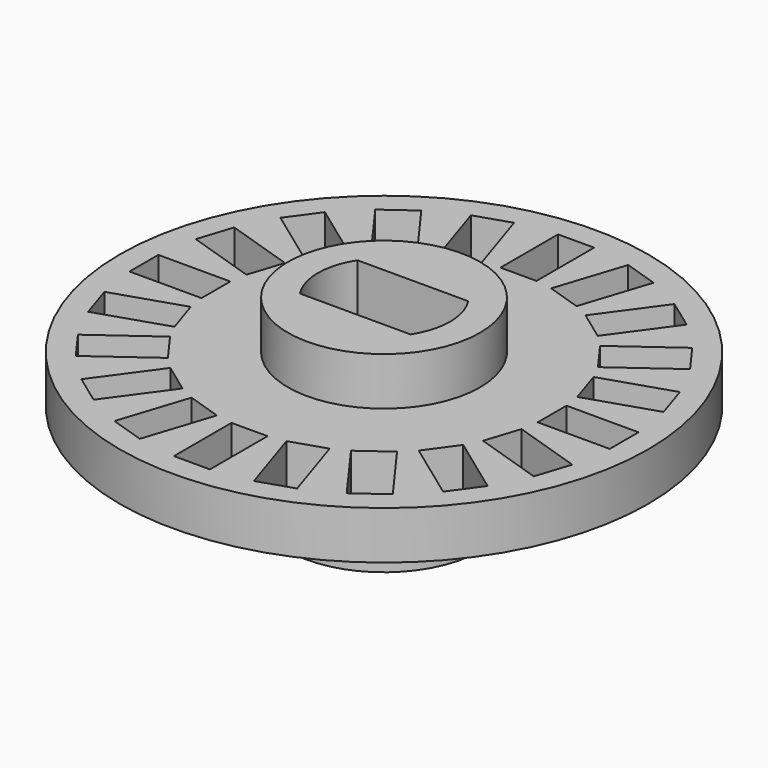
from build123d import *

# Parameters (mm, degrees)
F0_R            = 11
F1_DEPTH        = 2
F2_W            = 3
F2_H            = 1.5
F3_DEPTH        = 2
F3_COPIES_COUNT = 20
F4_R            = 4
F5_DEPTH        = 4
F5_DEPTH_BACK   = 4
F7_DEPTH        = 9


# Not quite as in the source:
# - a pattern or mirror of a feature is missing from the dataset's text; its kind, count and spacing are read off the source's solid


with BuildPart() as f1:
    # F0 (on Top) → F1 (new body)
    with BuildSketch(Plane.XY):
        Circle(F0_R)
    extrude(amount=F1_DEPTH)

    # F2 (on face) → F3 (cut)
    with BuildSketch(Plane.XY.offset(2)):
        with Locations((8.5, 0)):
            Rectangle(F2_W, F2_H)
    f3 = extrude(amount=-F3_DEPTH, mode=Mode.SUBTRACT)

    # F3_copies: F3 ×20 about axis
    f3_copies_axis = Axis((0, 0, 0), (0, 0, 1))
    for i in range(1, F3_COPIES_COUNT):
        add(f3.rotate(f3_copies_axis, i * 360 / F3_COPIES_COUNT), mode=Mode.SUBTRACT)

    # F4 (on face) → F5 (join, two sides)
    with BuildSketch(Plane(origin=(0, 0, 0), x_dir=(1, 0, 0), z_dir=(0, 0, -1))) as f5_sk:
        Circle(F4_R)
    extrude(amount=F5_DEPTH)
    extrude(f5_sk.sketch, amount=-F5_DEPTH_BACK)

    # F6 (on face) → F7 (cut)
    with BuildSketch(Plane.XY.offset(4)):
        with BuildLine():
            Line((-2.3048861143, -1.5), (2.3048861143, -1.5))
            ThreePointArc((2.3048861143, -1.5), (2.75, 0), (2.3048861143, 1.5))
            Line((2.3048861143, 1.5), (-2.3048861143, 1.5))
            ThreePointArc((-2.3048861143, 1.5), (-2.75, 0), (-2.3048861143, -1.5))
        make_face()
    extrude(amount=-F7_DEPTH, mode=Mode.SUBTRACT)


solid = f1.part
